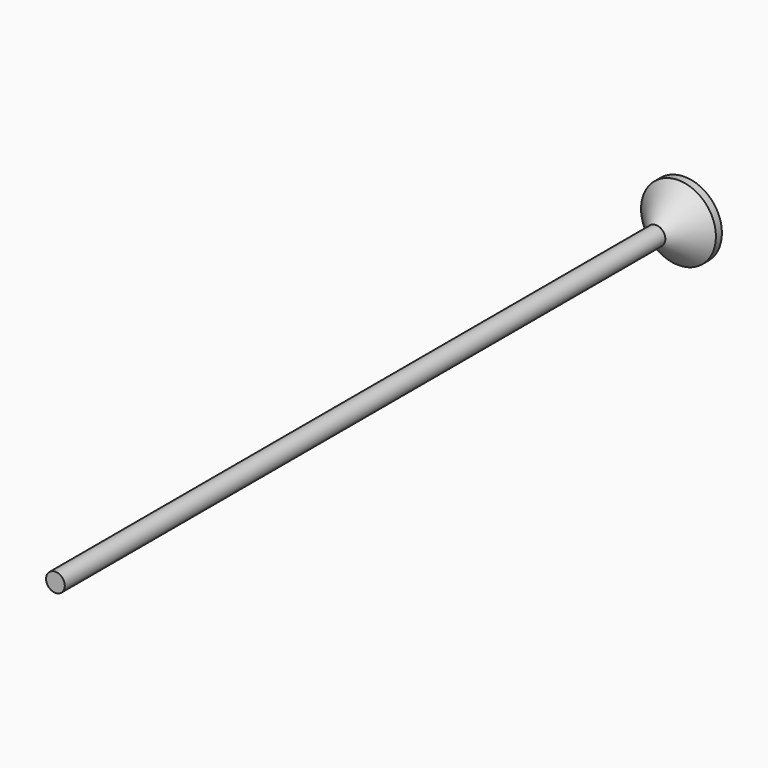
from build123d import *

# Parameters (mm, degrees)
F0_R        = 5
F1_DEPTH    = 5
F2_R        = 1.25
F3_DEPTH    = 100
F4_S5_R     = 1.25
F4_T6_DEPTH = 9


# Not quite as in the source:
# - a fillet or chamfer that OpenCascade refuses, or shapes differently, is made with other operations: its cross-section is extruded or revolved along the edge and cut away or added


with BuildPart() as f1:
    # F0 (on Front) → F1 (new body)
    with BuildSketch(Plane.XZ):
        Circle(F0_R)
    extrude(amount=F1_DEPTH)

    # F2 (on face) → F3 (join)
    with BuildSketch(Plane.XZ.offset(5)):
        Circle(F2_R)
    extrude(amount=F3_DEPTH)

    # F4: chamfer of 4 on 1 edges, made by hand


with BuildPart() as f4_tool2:
    # F4_s3 → F4_t4 (revolve)
    with BuildSketch(Plane.XY):
        Polygon((5, -1), (1, -5), (5, -5), align=None)
    revolve(axis=Axis((0, -5, 0), (0, -1, 0)))

    # F4_s5 → F4_t6 (cut, symmetric)
    with BuildSketch(Plane.XZ.offset(3)):
        Circle(F4_S5_R)
    extrude(amount=F4_T6_DEPTH, both=True, mode=Mode.SUBTRACT)


with BuildPart() as f1_1:
    add(f1.part)

    # F4_t1: cut F4_tool2
    add(f4_tool2.part, mode=Mode.SUBTRACT)


solid = f1_1.part
